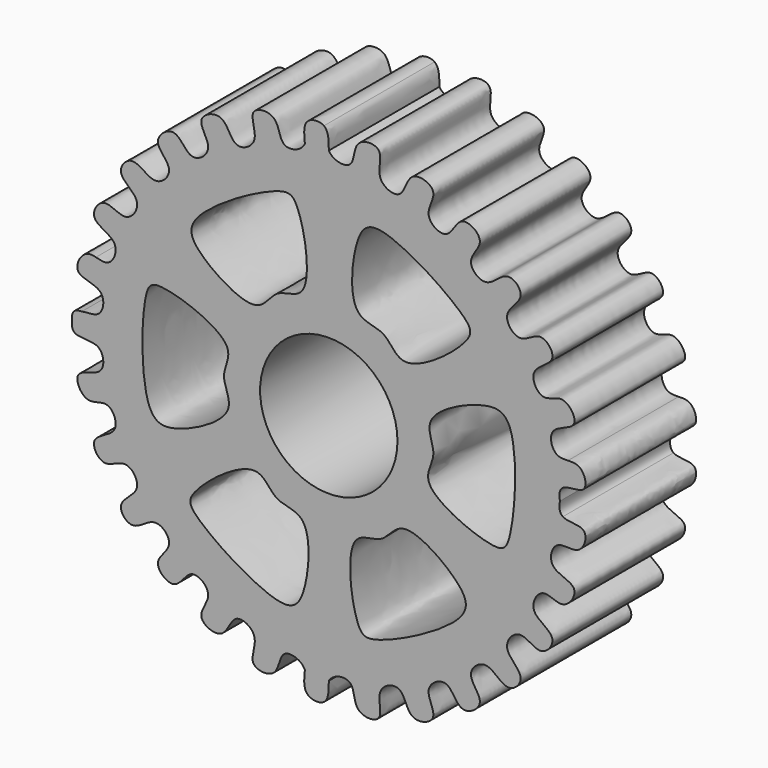
from build123d import *

# Parameters (mm, degrees)
F0_R     = 19.8638881117
F1_DEPTH = 40


with BuildPart() as f1:
    # F0 (on Front) → F1 (new body)
    with BuildSketch(Plane.XZ):
        with BuildLine():
            add(Edge.make_bspline(
                [(-1.414339873, 73.3596011996), (-0.0126052579, 72.3446225568), (-0.006302629, 69.9219268128), (0, 67.4992310689)],
                knots=[0.6534819585, 0.6534819585, 0.6534819585, 0.6534819585, 1, 1, 1, 1], degree=3))
            add(Edge.make_bspline(
                [(-1.414339873, 73.3596011996), (-1.1554982443, 71.0555180717), (-0.9209059484, 68.9672907887), (0, 67.4992310689)],
                knots=[0, 0, 0, 0, 0.0274302645, 0.0274302645, 0.0274302645, 0.0274302645], degree=3))
        make_face()
        with BuildLine():
            add(Edge.make_bspline(
                [(-1.414339873, 73.3596011996), (-1.1554982443, 71.0555180717), (-0.9209059484, 68.9672907887), (0, 67.4992310689)],
                knots=[0, 0, 0, 0, 0.0274302645, 0.0274302645, 0.0274302645, 0.0274302645], degree=3))
            add(Edge.make_bspline(
                [(-6.1281117394, 72.9577398026), (-4.9928445984, 74.0531594885), (-2.6560701629, 74.2587226959), (-1.414339873, 73.3596011996)],
                knots=[0.3465180415, 0.3465180415, 0.3465180415, 0.3465180415, 0.6534819585, 0.6534819585, 0.6534819585, 0.6534819585], degree=3))
            add(Edge.make_bspline(
                [(-6.1281117394, 72.9577398026), (-6.1402101228, 70.6391946384), (-6.1511750807, 68.5378601813), (-6.9105716062, 66.9801105147)],
                knots=[0, 0, 0, 0, 0.0274302645, 0.0274302645, 0.0274302645, 0.0274302645], degree=3))
            add(Edge.make_bspline(
                [(-6.9105716062, 66.9801105147), (-7.1325799433, 66.5247049374), (-8.4835202532, 64.5928484515), (-14.4870070711, 63.2534979205), (-14.1879747681, 72.3077342202), (-24.4400185643, 71.3502997788), (-19.1597700578, 62.7304461152), (-27.9494969626, 57.9699968587), (-29.7725927098, 68.0430611195), (-39.7317760064, 63.6432371786), (-32.3144922678, 56.8386818109), (-40.4008385467, 50.5759429012), (-43.906046867, 60.2020666645), (-52.2339794732, 53.3428815023), (-43.7350078393, 48.2370997082), (-50.3816423553, 41.0114471708), (-56.5909416642, 48.8395328556), (-62.5505947521, 41.4918514663), (-53.0545647466, 37.4212660505), (-58.5378177112, 29.1226090794), (-65.099825493, 35.4920736236), (-70.2940185353, 27.060613644), (-59.6523967753, 25.141370627), (-62.9361951469, 17.1243068416), (-66.1583738895, 18.1774353805), (-67.3437823964, 18.4463122007)],
                knots=[0.0274302645, 0.0274302645, 0.0274302645, 0.0274302645, 0.0354494576, 0.0653127808, 0.0985819168, 0.1299229711, 0.1644343925, 0.1959393351, 0.2305423939, 0.2625719527, 0.2966337575, 0.3281761578, 0.3622741999, 0.3940100821, 0.4280355371, 0.4591971764, 0.4945053127, 0.524035091, 0.5595487711, 0.5910370212, 0.624387296, 0.6546112062, 0.6903297873, 0.7218055012, 0.7400370629, 0.7400370629, 0.7400370629, 0.7400370629], degree=3))
            add(Edge.make_bspline(
                [(-66.5814855976, 10.4358245629), (-67.0826015045, 13.5489837138), (-67.8311958219, 16.9004175595), (-67.3437823964, 18.4463122007)],
                knots=[0.9677894695, 0.9677894695, 0.9677894695, 0.9677894695, 0.9911140979, 0.9911140979, 0.9911140979, 0.9911140979], degree=3))
            add(Edge.make_bspline(
                [(-66.5814855976, 10.4358245629), (-66.390426796, 10.3015893334), (-64.6076641114, 8.7795851079), (-65.1269226592, 5.2536920853), (-66.8062478006, 4.1556510146), (-66.8799923895, 4.1122430168)],
                knots=[0.8168221007, 0.8168221007, 0.8168221007, 0.8168221007, 0.8202112238, 0.8515310831, 0.8529284423, 0.8529284423, 0.8529284423, 0.8529284423], degree=3))
            add(Edge.make_bspline(
                [(-71.4580757748, 3.281939848), (-69.8230599254, 3.3275005182), (-67.862680171, 3.0749603426), (-66.8799923895, 4.1122430168)],
                knots=[0.9255246506, 0.9255246506, 0.9255246506, 0.9255246506, 0.9469629485, 0.9469629485, 0.9469629485, 0.9469629485], degree=3))
            add(Edge.make_bspline(
                [(-71.4580757756, 3.2819398543), (-71.9644520267, 3.1611527998), (-73.296438606, 2.6208803571), (-74.0741998892, 1.0284556597), (-74.2469210996, 0)],
                knots=[0.8765448361, 0.8765448361, 0.8765448361, 0.8765448361, 0.8844732145, 0.898972482, 0.898972482, 0.898972482, 0.898972482], degree=3))
            add(Edge.make_bspline(
                [(-71.4580758055, -3.2819398471), (-71.9644520452, -3.1611527923), (-73.2964386114, -2.620880346), (-74.0741998892, -1.0284556597), (-74.2469210996, 0)],
                knots=[0.8765448363, 0.8765448363, 0.8765448363, 0.8765448363, 0.8844732145, 0.898972482, 0.898972482, 0.898972482, 0.898972482], degree=3))
            add(Edge.make_bspline(
                [(-71.4580758055, -3.2819398471), (-69.8230599499, -3.3275005214), (-67.8626801771, -3.0749603361), (-66.8799923895, -4.1122430168)],
                knots=[0.9255246504, 0.9255246504, 0.9255246504, 0.9255246504, 0.9469629485, 0.9469629485, 0.9469629485, 0.9469629485], degree=3))
            add(Edge.make_bspline(
                [(-66.5814856051, -10.4358245682), (-66.3904268005, -10.3015893373), (-64.6076641108, -8.7795851123), (-65.1269226592, -5.2536920853), (-66.8062478006, -4.1556510146), (-66.8799923895, -4.1122430168)],
                knots=[0.8168221007, 0.8168221007, 0.8168221007, 0.8168221007, 0.8202112238, 0.8515310831, 0.8529284423, 0.8529284423, 0.8529284423, 0.8529284423], degree=3))
            add(Edge.make_bspline(
                [(-66.581485599, -10.4358245714), (-67.0826015059, -13.5489837205), (-67.8311958217, -16.900417562), (-67.3437823962, -18.4463122015)],
                knots=[0.9677894695, 0.9677894695, 0.9677894695, 0.9677894695, 0.9911140979, 0.9911140979, 0.9911140979, 0.9911140979], degree=3))
            add(Edge.make_bspline(
                [(-6.9105716062, -66.9801105147), (-7.1325799433, -66.5247049374), (-8.4835202532, -64.5928484515), (-14.4870070711, -63.2534979205), (-14.1879747681, -72.3077342202), (-24.4400185643, -71.3502997788), (-19.1597700578, -62.7304461152), (-27.9494969626, -57.9699968587), (-29.7725927098, -68.0430611195), (-39.7317760064, -63.6432371786), (-32.3144922678, -56.8386818109), (-40.4008385467, -50.5759429012), (-43.906046867, -60.2020666645), (-52.2339794732, -53.3428815023), (-43.7350078393, -48.2370997082), (-50.3816423553, -41.0114471708), (-56.5909416642, -48.8395328556), (-62.5505947521, -41.4918514663), (-53.0545647466, -37.4212660505), (-58.5378177112, -29.1226090794), (-65.099825493, -35.4920736236), (-70.2940185353, -27.060613644), (-59.6523967753, -25.141370627), (-62.9361951459, -17.1243068438), (-66.1583738864, -18.1774353795), (-67.3437823917, -18.4463121997)],
                knots=[0.0274302645, 0.0274302645, 0.0274302645, 0.0274302645, 0.0354494576, 0.0653127808, 0.0985819168, 0.1299229711, 0.1644343925, 0.1959393351, 0.2305423939, 0.2625719527, 0.2966337575, 0.3281761578, 0.3622741999, 0.3940100821, 0.4280355371, 0.4591971764, 0.4945053127, 0.524035091, 0.5595487711, 0.5910370212, 0.624387296, 0.6546112062, 0.6903297873, 0.7218055012, 0.7400370629, 0.7400370629, 0.7400370629, 0.7400370629], degree=3))
            add(Edge.make_bspline(
                [(-6.1281117394, -72.9577398026), (-6.1402101228, -70.6391946384), (-6.1511750807, -68.5378601813), (-6.9105716062, -66.9801105147)],
                knots=[0, 0, 0, 0, 0.0274302645, 0.0274302645, 0.0274302645, 0.0274302645], degree=3))
            add(Edge.make_bspline(
                [(-6.1281117394, -72.9577398026), (-4.9928445984, -74.0531594885), (-2.6560701629, -74.2587226959), (-1.414339873, -73.3596011996)],
                knots=[0.3465180415, 0.3465180415, 0.3465180415, 0.3465180415, 0.6534819585, 0.6534819585, 0.6534819585, 0.6534819585], degree=3))
            add(Edge.make_bspline(
                [(-1.414339873, -73.3596011996), (-1.1554982443, -71.0555180717), (-0.9209059484, -68.9672907887), (0, -67.4992310689)],
                knots=[0, 0, 0, 0, 0.0274302645, 0.0274302645, 0.0274302645, 0.0274302645], degree=3))
            add(Edge.make_bspline(
                [(0, -67.4992310689), (0.2692253538, -67.0700462014), (1.8181380219, -65.29297593), (7.9300880892, -64.6003142577), (6.6689203014, -73.5712713471), (16.9646312877, -73.7106198131), (12.6319795934, -64.5776558491), (21.8785182955, -60.7799330821), (22.6189649747, -70.9898322207), (32.9899261201, -67.6751757427), (26.3391412489, -60.1197053796), (35.0462165714, -54.7533533483), (37.5067952998, -64.6979144948), (46.5175766761, -58.7642224257), (38.610413602, -52.7827260675), (45.9884610542, -46.3056726655), (51.329169291, -54.7502661385), (58.037128917, -48.0787472423), (49.0283749024, -43.0204271065), (55.3638738688, -35.3526227634), (61.2105584798, -42.3844293426), (67.272777028, -34.5538058029), (56.8959275488, -31.5126543226), (61.6733731069, -22.6713653388), (67.9420946861, -28.383996216), (73.6521734514, -19.4510290731), (62.7849942417, -18.7889992006), (64.8215763897, -10.9076052327), (68.0580191651, -11.0345815423), (69.1701498773, -11.0706562451)],
                knots=[0.0274302645, 0.0274302645, 0.0274302645, 0.0274302645, 0.0354494576, 0.0653127808, 0.0985819168, 0.1299229711, 0.1644343925, 0.1959393351, 0.2305423939, 0.2625719527, 0.2966337575, 0.3281761578, 0.3622741999, 0.3940100821, 0.4280355371, 0.4591971764, 0.4945053127, 0.524035091, 0.5595487711, 0.5910370212, 0.624387296, 0.6546112062, 0.6903297873, 0.7218055012, 0.7537033149, 0.7852457194, 0.8202112238, 0.8515310831, 0.8677153511, 0.8677153511, 0.8677153511, 0.8677153511], degree=3))
            add(Edge.make_bspline(
                [(67.7257783755, -3.6777736161), (68.5416527675, -6.5940757347), (69.5111603098, -9.5987996568), (69.1701498789, -11.0706562457)],
                knots=[0.9691979475, 0.9691979475, 0.9691979475, 0.9691979475, 0.9914220002, 0.9914220002, 0.9914220002, 0.9914220002], degree=3))
            add(Edge.make_bspline(
                [(67.7257783754, -3.6777736162), (67.3508638008, -3.4348909405), (66.653740583, -2.6347071495), (66.6945567212, -1.0599354754), (66.8599998872, 0)],
                knots=[0.943328918, 0.943328918, 0.943328918, 0.943328918, 0.9500228296, 0.959367335, 0.959367335, 0.959367335, 0.959367335], degree=3))
            add(Edge.make_bspline(
                [(67.7257783756, 3.6777736163), (67.3508638009, 3.4348909406), (66.653740583, 2.6347071496), (66.6945567212, 1.0599354754), (66.8599998872, 0)],
                knots=[0.943328918, 0.943328918, 0.943328918, 0.943328918, 0.9500228296, 0.959367335, 0.959367335, 0.959367335, 0.959367335], degree=3))
            add(Edge.make_bspline(
                [(67.7257783756, 3.6777736163), (68.5416527679, 6.594075736), (69.5111603106, 9.5987996591), (69.1701498785, 11.0706562474)],
                knots=[0.9691979475, 0.9691979475, 0.9691979475, 0.9691979475, 0.9914220002, 0.9914220002, 0.9914220002, 0.9914220002], degree=3))
            add(Edge.make_bspline(
                [(0, 67.4992310689), (0.2692253538, 67.0700462014), (1.8181380219, 65.29297593), (7.9300880892, 64.6003142577), (6.6689203014, 73.5712713471), (16.9646312877, 73.7106198131), (12.6319795934, 64.5776558491), (21.8785182955, 60.7799330821), (22.6189649747, 70.9898322207), (32.9899261201, 67.6751757427), (26.3391412489, 60.1197053796), (35.0462165714, 54.7533533483), (37.5067952998, 64.6979144948), (46.5175766761, 58.7642224257), (38.610413602, 52.7827260675), (45.9884610542, 46.3056726655), (51.329169291, 54.7502661385), (58.037128917, 48.0787472423), (49.0283749024, 43.0204271065), (55.3638738688, 35.3526227634), (61.2105584798, 42.3844293426), (67.272777028, 34.5538058029), (56.8959275488, 31.5126543226), (61.6733731069, 22.6713653388), (67.9420946861, 28.383996216), (73.6521734514, 19.4510290731), (62.7849942417, 18.7889992006), (64.8215763898, 10.9076052324), (68.0580191656, 11.0345815424), (69.1701498781, 11.0706562451)],
                knots=[0.0274302645, 0.0274302645, 0.0274302645, 0.0274302645, 0.0354494576, 0.0653127808, 0.0985819168, 0.1299229711, 0.1644343925, 0.1959393351, 0.2305423939, 0.2625719527, 0.2966337575, 0.3281761578, 0.3622741999, 0.3940100821, 0.4280355371, 0.4591971764, 0.4945053127, 0.524035091, 0.5595487711, 0.5910370212, 0.624387296, 0.6546112062, 0.6903297873, 0.7218055012, 0.7537033149, 0.7852457194, 0.8202112238, 0.8515310831, 0.8677153511, 0.8677153511, 0.8677153511, 0.8677153511], degree=3))
        make_face()
        with BuildLine():
            add(Edge.make_bspline(
                [(-21.4063283056, -21.0088342428), (-26.2626612991, -20.6734681935), (-41.0218892224, -32.1730724993), (-39.8394478175, -38.6028153928), (-12.8791249937, -56.0495244012), (-6.0800704277, -47.7195280117), (-4.5119030034, -26.3001844652), (-16.1826514242, -27.6922856822), (-18.4197987232, -21.2150764071), (-21.4063283056, -21.0088342428)],
                knots=[0, 0, 0, 0, 0.1836282822, 0.2762927883, 0.4907691742, 0.6041784726, 0.7730914255, 0.8870729627, 1, 1, 1, 1], degree=3))
        make_face(mode=Mode.SUBTRACT)
        with BuildLine():
            add(Edge.make_bspline(
                [(-29.5496582985, 8.1854965538), (-31.8486103003, 12.4763309976), (-49.436781133, 18.8584901027), (-54.2527383896, 14.4373684062), (-54.6875972568, -17.67271661), (-44.017323079, -18.9998307011), (-25.0448299806, -8.9354413672), (-32.4310416297, 0.2072164507), (-28.1358573563, 5.5467351639), (-29.5496582985, 8.1854965538)],
                knots=[0, 0, 0, 0, 0.1836282822, 0.2762927883, 0.4907691742, 0.6041784726, 0.7730914255, 0.8870729627, 1, 1, 1, 1], degree=3))
        make_face(mode=Mode.SUBTRACT)
        Circle(F0_R, mode=Mode.SUBTRACT)
        with BuildLine():
            add(Edge.make_bspline(
                [(7.6567828655, -29.4489916414), (4.9004835314, -33.4613792736), (7.3061548331, -52.016390825), (13.4449085819, -54.2648266734), (42.1700738876, -39.9082414197), (38.4499288224, -29.8198072729), (20.7981117142, -17.5862150036), (16.0673622722, -28.3455980815), (9.3518415673, -26.9814684349), (7.6567828655, -29.4489916414)],
                knots=[0, 0, 0, 0, 0.1836282822, 0.2762927883, 0.4907691742, 0.6041784726, 0.7730914255, 0.8870729627, 1, 1, 1, 1], degree=3))
        make_face(mode=Mode.SUBTRACT)
        with BuildLine():
            add(Edge.make_bspline(
                [(29.1269179434, -7.8856293112), (31.2235978956, -12.2788483711), (48.4955449175, -19.4729816864), (53.5121243554, -15.2808829165), (55.4415394669, 16.7741325929), (44.8446266788, 18.5966095341), (25.4241164399, 9.4264836302), (32.3766407935, -0.0501571045), (27.837509513, -5.1839038113), (29.1269179434, -7.8856293112)],
                knots=[0, 0, 0, 0, 0.1836282822, 0.2762927883, 0.4907691742, 0.6041784726, 0.7730914255, 0.8870729627, 1, 1, 1, 1], degree=3))
        make_face(mode=Mode.SUBTRACT)
        with BuildLine():
            add(Edge.make_bspline(
                [(-7.5072608888, 29.6082664281), (-4.9307079497, 33.7383772599), (-8.1528439056, 52.1691544536), (-14.3848381218, 54.1445049143), (-42.4484838387, 38.5343014865), (-38.286773473, 28.6198600159), (-20.1122995354, 17.1771363835), (-15.8609558763, 28.1347999845), (-9.0917798219, 27.0683462468), (-7.5072608888, 29.6082664281)],
                knots=[0, 0, 0, 0, 0.1836282822, 0.2762927883, 0.4907691742, 0.6041784726, 0.7730914255, 0.8870729627, 1, 1, 1, 1], degree=3))
        make_face(mode=Mode.SUBTRACT)
        with BuildLine():
            add(Edge.make_bspline(
                [(22.1408400685, 20.9393072873), (26.9938193549, 20.5584758597), (41.860095075, 31.9193540958), (40.7379207641, 38.359888714), (13.94217057, 56.0583189698), (7.065402847, 47.7923617642), (5.2967097163, 26.3886435909), (16.9799835119, 27.6713859341), (19.1563729364, 21.1735095808), (22.1408400685, 20.9393072873)],
                knots=[0, 0, 0, 0, 0.1836282822, 0.2762927883, 0.4907691742, 0.6041784726, 0.7730914255, 0.8870729627, 1, 1, 1, 1], degree=3))
        make_face(mode=Mode.SUBTRACT)
        with BuildLine():
            add(Edge.make_bspline(
                [(-6.1281117394, 72.9577398026), (-6.1402101228, 70.6391946384), (-6.1511750807, 68.5378601813), (-6.9105716062, 66.9801105147)],
                knots=[0, 0, 0, 0, 0.0274302645, 0.0274302645, 0.0274302645, 0.0274302645], degree=3))
            add(Edge.make_bspline(
                [(-6.9105716062, 66.9801105147), (-7.1601182013, 69.3506396484), (-7.4096647964, 71.7211687821), (-6.1281117394, 72.9577398026)],
                knots=[0, 0, 0, 0, 0.3465180415, 0.3465180415, 0.3465180415, 0.3465180415], degree=3))
        make_face()
        with BuildLine():
            add(Edge.make_bspline(
                [(69.1701498781, 11.0706562451), (70.321696218, 11.1080094909), (73.6047199375, 11.1917990627), (75.7208425888, 3.4578691643), (69.3083669738, 4.7030294457), (67.7257783756, 3.6777736163)],
                knots=[0.8677153511, 0.8677153511, 0.8677153511, 0.8677153511, 0.8844732145, 0.9150725929, 0.943328918, 0.943328918, 0.943328918, 0.943328918], degree=3))
            add(Edge.make_bspline(
                [(67.7257783756, 3.6777736163), (68.5416527679, 6.594075736), (69.5111603106, 9.5987996591), (69.1701498785, 11.0706562474)],
                knots=[0.9691979475, 0.9691979475, 0.9691979475, 0.9691979475, 0.9914220002, 0.9914220002, 0.9914220002, 0.9914220002], degree=3))
        make_face()
        with BuildLine():
            add(Edge.make_bspline(
                [(-66.5814855976, 10.4358245629), (-67.0826015045, 13.5489837138), (-67.8311958219, 16.9004175595), (-67.3437823964, 18.4463122007)],
                knots=[0.9677894695, 0.9677894695, 0.9677894695, 0.9677894695, 0.9911140979, 0.9911140979, 0.9911140979, 0.9911140979], degree=3))
            add(Edge.make_bspline(
                [(-67.3437823964, 18.4463122007), (-68.2323563758, 18.6478603967), (-71.1784633028, 19.0963957492), (-74.866668282, 11.6913977849), (-68.3615760197, 11.686491082), (-66.5814855976, 10.4358245629)],
                knots=[0.7400370629, 0.7400370629, 0.7400370629, 0.7400370629, 0.7537033149, 0.7852457194, 0.8168221007, 0.8168221007, 0.8168221007, 0.8168221007], degree=3))
        make_face()
        with BuildLine():
            add(Edge.make_bspline(
                [(69.1701498773, -11.0706562451), (70.3216962174, -11.1080094909), (73.6047199374, -11.1917990632), (75.7208425888, -3.4578691642), (69.3083669736, -4.7030294457), (67.7257783754, -3.6777736162)],
                knots=[0.8677153511, 0.8677153511, 0.8677153511, 0.8677153511, 0.8844732145, 0.9150725929, 0.943328918, 0.943328918, 0.943328918, 0.943328918], degree=3))
            add(Edge.make_bspline(
                [(67.7257783755, -3.6777736161), (68.5416527675, -6.5940757347), (69.5111603098, -9.5987996568), (69.1701498789, -11.0706562457)],
                knots=[0.9691979475, 0.9691979475, 0.9691979475, 0.9691979475, 0.9914220002, 0.9914220002, 0.9914220002, 0.9914220002], degree=3))
        make_face()
        with BuildLine():
            add(Edge.make_bspline(
                [(-71.4580757748, 3.281939848), (-69.8230599254, 3.3275005182), (-67.862680171, 3.0749603426), (-66.8799923895, 4.1122430168)],
                knots=[0.9255246506, 0.9255246506, 0.9255246506, 0.9255246506, 0.9469629485, 0.9469629485, 0.9469629485, 0.9469629485], degree=3))
            add(Edge.make_bspline(
                [(-66.8799923895, 4.1122430168), (-68.1263299223, 3.3786160786), (-69.9497243347, 3.6417302814), (-71.4580757756, 3.2819398543)],
                knots=[0.8529284423, 0.8529284423, 0.8529284423, 0.8529284423, 0.8765448361, 0.8765448361, 0.8765448361, 0.8765448361], degree=3))
        make_face()
        with BuildLine():
            add(Edge.make_bspline(
                [(-71.4580757756, 3.2819398543), (-71.9644520267, 3.1611527998), (-73.296438606, 2.6208803571), (-74.0741998892, 1.0284556597), (-74.2469210996, 0)],
                knots=[0.8765448361, 0.8765448361, 0.8765448361, 0.8765448361, 0.8844732145, 0.898972482, 0.898972482, 0.898972482, 0.898972482], degree=3))
            add(Edge.make_bspline(
                [(-74.2469210996, 0), (-74.4387122113, 1.1420059751), (-74.0837771907, 3.0232935369), (-72.2552136859, 3.2597271352), (-71.4580757748, 3.281939848)],
                knots=[0.898972482, 0.898972482, 0.898972482, 0.898972482, 0.9150725929, 0.9255246506, 0.9255246506, 0.9255246506, 0.9255246506], degree=3))
        make_face()
        with BuildLine():
            add(Edge.make_bspline(
                [(-1.414339873, -73.3596011996), (-0.0126052579, -72.3446225568), (-0.006302629, -69.9219268128), (0, -67.4992310689)],
                knots=[0.6534819585, 0.6534819585, 0.6534819585, 0.6534819585, 1, 1, 1, 1], degree=3))
            add(Edge.make_bspline(
                [(-1.414339873, -73.3596011996), (-1.1554982443, -71.0555180717), (-0.9209059484, -68.9672907887), (0, -67.4992310689)],
                knots=[0, 0, 0, 0, 0.0274302645, 0.0274302645, 0.0274302645, 0.0274302645], degree=3))
        make_face()
        with BuildLine():
            add(Edge.make_bspline(
                [(-71.4580758055, -3.2819398471), (-71.9644520452, -3.1611527923), (-73.2964386114, -2.620880346), (-74.0741998892, -1.0284556597), (-74.2469210996, 0)],
                knots=[0.8765448363, 0.8765448363, 0.8765448363, 0.8765448363, 0.8844732145, 0.898972482, 0.898972482, 0.898972482, 0.898972482], degree=3))
            add(Edge.make_bspline(
                [(-74.2469210996, 0), (-74.4387122113, -1.1420059751), (-74.0837771925, -3.0232935274), (-72.2552137044, -3.2597271328), (-71.4580758055, -3.2819398471)],
                knots=[0.898972482, 0.898972482, 0.898972482, 0.898972482, 0.9150725929, 0.9255246504, 0.9255246504, 0.9255246504, 0.9255246504], degree=3))
        make_face()
        with BuildLine():
            add(Edge.make_bspline(
                [(-71.4580758055, -3.2819398471), (-69.8230599499, -3.3275005214), (-67.8626801771, -3.0749603361), (-66.8799923895, -4.1122430168)],
                knots=[0.9255246504, 0.9255246504, 0.9255246504, 0.9255246504, 0.9469629485, 0.9469629485, 0.9469629485, 0.9469629485], degree=3))
            add(Edge.make_bspline(
                [(-66.8799923895, -4.1122430168), (-68.1263299306, -3.3786160737), (-69.9497243587, -3.6417302849), (-71.4580758055, -3.2819398471)],
                knots=[0.8529284423, 0.8529284423, 0.8529284423, 0.8529284423, 0.8765448363, 0.8765448363, 0.8765448363, 0.8765448363], degree=3))
        make_face()
        with BuildLine():
            add(Edge.make_bspline(
                [(-6.9105716062, -66.9801105147), (-7.1601182013, -69.3506396484), (-7.4096647964, -71.7211687821), (-6.1281117394, -72.9577398026)],
                knots=[0, 0, 0, 0, 0.3465180415, 0.3465180415, 0.3465180415, 0.3465180415], degree=3))
            add(Edge.make_bspline(
                [(-6.1281117394, -72.9577398026), (-6.1402101228, -70.6391946384), (-6.1511750807, -68.5378601813), (-6.9105716062, -66.9801105147)],
                knots=[0, 0, 0, 0, 0.0274302645, 0.0274302645, 0.0274302645, 0.0274302645], degree=3))
        make_face()
        with BuildLine():
            add(Edge.make_bspline(
                [(-66.581485599, -10.4358245714), (-67.0826015059, -13.5489837205), (-67.8311958217, -16.900417562), (-67.3437823962, -18.4463122015)],
                knots=[0.9677894695, 0.9677894695, 0.9677894695, 0.9677894695, 0.9911140979, 0.9911140979, 0.9911140979, 0.9911140979], degree=3))
            add(Edge.make_bspline(
                [(-67.3437823917, -18.4463121997), (-68.2323563726, -18.6478603963), (-71.1784633016, -19.0963957515), (-74.8666682798, -11.6913977892), (-68.3615760289, -11.686491082), (-66.5814856051, -10.4358245682)],
                knots=[0.7400370629, 0.7400370629, 0.7400370629, 0.7400370629, 0.7537033149, 0.7852457194, 0.8168221007, 0.8168221007, 0.8168221007, 0.8168221007], degree=3))
        make_face()
    extrude(amount=F1_DEPTH)


solid = f1.part
